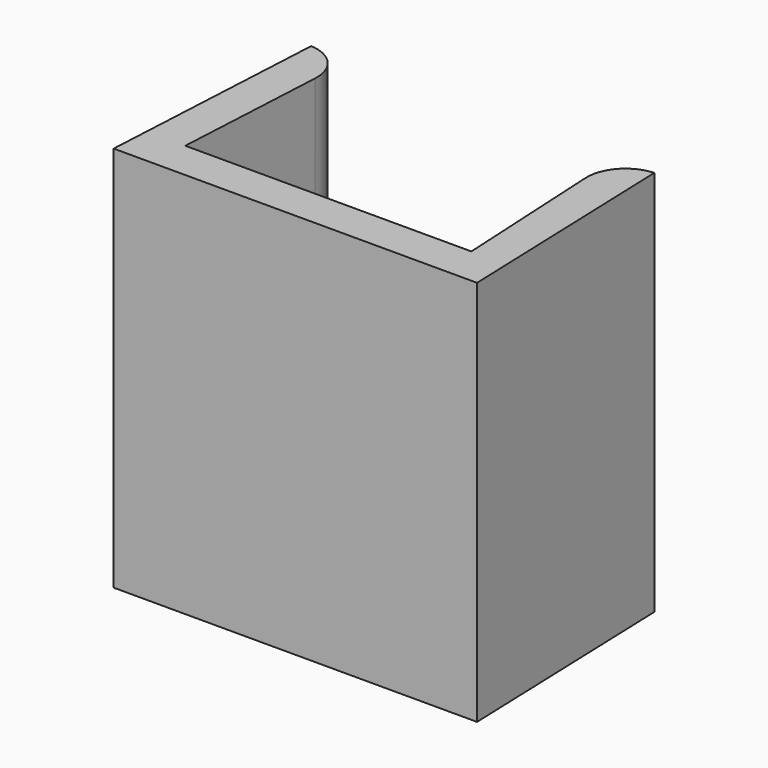
from build123d import *

# Parameters (mm, degrees)
F1_DEPTH    = 10
F2_T1_DEPTH = 15.2616750858


# Not quite as in the source:
# - a fillet or chamfer that OpenCascade refuses, or shapes differently, is made with other operations: its cross-section is extruded or revolved along the edge and cut away or added


with BuildPart() as f1:
    # F0 (on Top) → F1 (new body)
    with BuildSketch(Plane.XY):
        Polygon((4.7359447583, 0), (-2.6640552417, 0), (-2.4023754605, 4.9931476738), (-3.4023754605, 4.9931476738), (-3.716463021, -1), (5.683536979, -1), (5.474264977, 4.9931476738), (4.474264977, 4.9931476738), align=None)
    extrude(amount=F1_DEPTH)

    # F2: fillet of radius 1 on 2 edges, made by hand

    # F2_s2 → F2_t1 (cut)
    with BuildSketch(Plane.XY.offset(-2.6308375429)):
        with BuildLine():
            ThreePointArc((5.474264977, 4.9931476738), (4.78436631, 4.6632120235), (4.5293399365, 3.9422548452))
            Line((4.5293399365, 3.9422548452), (4.474264977, 4.9931476738))
            Line((4.474264977, 4.9931476738), (5.474264977, 4.9931476738))
        make_face()
        with BuildLine():
            ThreePointArc((-2.4574504199, 3.9422548452), (-2.7124767935, 4.6632120235), (-3.4023754605, 4.9931476738))
            Line((-3.4023754605, 4.9931476738), (-2.4023754605, 4.9931476738))
            Line((-2.4023754605, 4.9931476738), (-2.4574504199, 3.9422548452))
        make_face()
    extrude(amount=F2_T1_DEPTH, mode=Mode.SUBTRACT)


solid = f1.part
